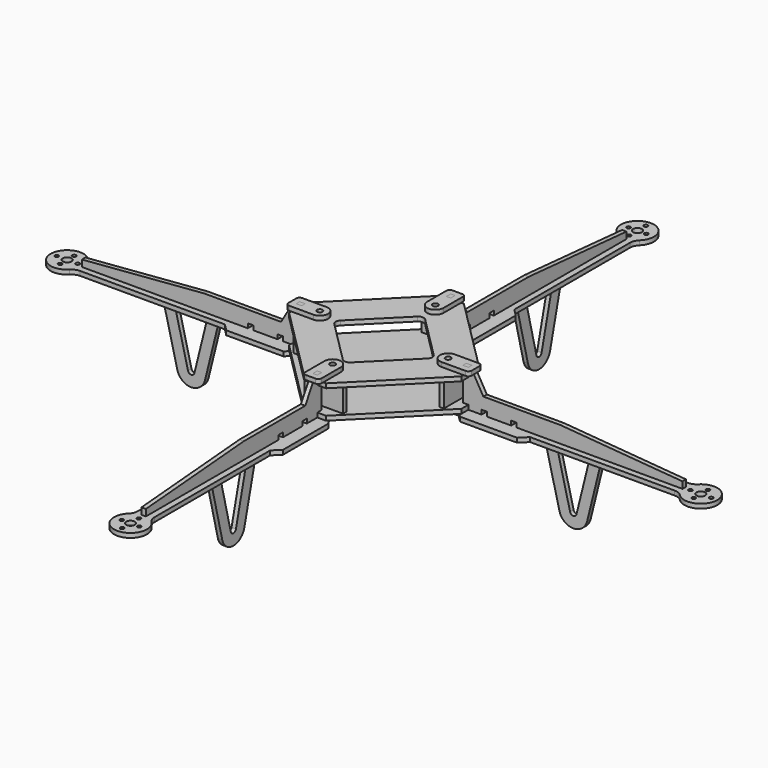
from build123d import *

# Parameters (mm, degrees)
F3_DEPTH  = 4
F7_DEPTH  = 25
F8_R      = 5
F9_R      = 2.5
F9_R_2    = 1.75
F9_R_3    = 4
F11_DEPTH = 4
F13_DEPTH = 2
F15_DEPTH = 2
F16_R     = 2.5
F17_DEPTH = 4
F20_W     = 35
F20_H     = 4
F21_DEPTH = 22
F22_COUNT = 4


# Not quite as in the source:
# - a feature names something its author has since deleted; it is built from what else it names


with BuildPart() as f3:
    # F2 (on Top) → F3 (new body)
    with BuildSketch(Plane.XY):
        Polygon((78.3883476483, 10), (10, 78.3883476483), (2, 78.3883476483), (2, 73.3883476483), (-2, 73.3883476483), (-2, 78.3883476483), (-10, 78.3883476483), (-78.3883476483, 10), (-78.3883476483, 2), (-73.3883476483, 2), (-73.3883476483, -2), (-78.3883476483, -2), (-78.3883476483, -10), (-10, -78.3883476483), (-2, -78.3883476483), (-2, -73.3883476483), (2, -73.3883476483), (2, -78.3883476483), (10, -78.3883476483), (78.3883476483, -10), (78.3883476483, -2), (73.3883476483, -2), (73.3883476483, 2), (78.3883476483, 2), align=None)
    extrude(amount=F3_DEPTH)


with BuildPart() as f5_1:
    # F5: copy of F3
    add(f3.part.moved(Location((0, 0, 26))))

    # F6 (on face) → F7 (cut)
    with BuildSketch(Plane.XY.offset(30)):
        Polygon((-45.9619407771, 0), (0, -45.9619407771), (45.9619407771, 0), (0, 45.9619407771), align=None)
    extrude(amount=-F7_DEPTH, mode=Mode.SUBTRACT)

    # F8
    f8_edges = [f5_1.edges().sort_by_distance(p)[0] for p in [
        (0, -45.961941, 28),
        (-45.961941, 0, 28),
        (0, 45.961941, 28),
        (45.961941, 0, 28),
    ]]
    fillet(f8_edges, radius=F8_R)


with BuildPart() as f11:
    # F9 (on Top) → F11 (new body)
    with BuildSketch(Plane.XY):
        with BuildLine():
            ThreePointArc((7.5, 270.534776577), (8.2804555427, 274.4077599232), (10.5, 277.6762050055))
            ThreePointArc((10.5, 277.6762050055), (0, 303.3883476483), (-10.5, 277.6762050055))
            ThreePointArc((-10.5, 277.6762050055), (-8.2804555427, 274.4077599232), (-7.5, 270.534776577))
            Line((-7.5, 270.534776577), (-7.5, 138.8883476483))
            Line((-7.5, 138.8883476483), (-14, 132.3883476483))
            Line((-14, 132.3883476483), (-14, 80.3883476483))
            Line((-14, 80.3883476483), (-7.5, 73.8883476483))
            Line((-7.5, 73.8883476483), (-7.5, 58.3883476483))
            ThreePointArc((-7.5, 58.3883476483), (0, 50.8883476483), (7.5, 58.3883476483))
            Line((7.5, 58.3883476483), (7.5, 73.8883476483))
            Line((7.5, 73.8883476483), (14, 80.3883476483))
            Line((14, 80.3883476483), (14, 132.3883476483))
            Line((14, 132.3883476483), (7.5, 138.8883476483))
            Line((7.5, 138.8883476483), (7.5, 270.534776577))
        make_face()
        with Locations((0, 58.3883476483)):
            Circle(F9_R, mode=Mode.SUBTRACT)
        with Locations((-8, 288.3883476483)):
            Circle(F9_R_2, mode=Mode.SUBTRACT)
        with Locations((0, 278.8883476483)):
            Circle(F9_R_2, mode=Mode.SUBTRACT)
        with Locations((0, 288.3883476483)):
            Circle(F9_R_3, mode=Mode.SUBTRACT)
        with Locations((0, 297.8883476483)):
            Circle(F9_R_2, mode=Mode.SUBTRACT)
        with Locations((8, 288.3883476483)):
            Circle(F9_R_2, mode=Mode.SUBTRACT)
    extrude(amount=-F11_DEPTH)


with BuildPart() as f13:
    # F12 (on Right) → F13 (new body, symmetric)
    with BuildSketch(Plane.YZ):
        Polygon((162.0486016862, 15), (92.0486016862, 15), (83.3883476483, 30), (78.3883476483, 30), (78.3883476483, 34), (73.3883476483, 34), (73.3883476483, 0), (80.3883476483, 0), (80.3883476483, -4), (90.3883476483, -4), (90.3883476483, 4), (95.3883476483, 4), (95.3883476483, 0), (117.3883476483, 0), (117.3883476483, 4), (122.3883476483, 4), (122.3883476483, 0), (263.3883476483, 0), (263.3883476483, -4), (273.3883476483, -4), (273.3883476483, 6), align=None)
    extrude(amount=F13_DEPTH, both=True)


with BuildPart() as f15:
    # F14 (on Right) → F15 (new body, symmetric)
    with BuildSketch(Plane.YZ):
        with BuildLine():
            Line((154.1888916965, -4), (148.8883476483, -4))
            Line((148.8883476483, -4), (161.2676550527, -54.1173896785))
            ThreePointArc((161.2676550527, -54.1173896785), (173.8883476483, -64), (186.5090402439, -54.1173896785))
            Line((186.5090402439, -54.1173896785), (198.8883476483, -4))
            Line((198.8883476483, -4), (193.5878036001, -4))
            Line((193.5878036001, -4), (193.5878036001, 0))
            Line((193.5878036001, 0), (188.5878036001, 0))
            Line((188.5878036001, 0), (188.5878036001, -4))
            Line((188.5878036001, -4), (176.8008151704, -51.7193976181))
            ThreePointArc((176.8008151704, -51.7193976181), (173.8883476483, -54), (170.9758801263, -51.7193976181))
            Line((170.9758801263, -51.7193976181), (159.1888916965, -4))
            Line((159.1888916965, -4), (159.1888916965, 0))
            Line((159.1888916965, 0), (154.1888916965, 0))
            Line((154.1888916965, 0), (154.1888916965, -4))
        make_face()
    extrude(amount=F15_DEPTH, both=True)


with BuildPart() as f17:
    # F16 (on offset) → F17 (new body)
    with BuildSketch(Plane.XY.offset(30)):
        with BuildLine():
            Line((-7.5, 80.3883476483), (-7.5, 73.8883476483))
            Line((-7.5, 73.8883476483), (-7.5, 58.3883476483))
            ThreePointArc((-7.5, 58.3883476483), (0, 50.8883476483), (7.5, 58.3883476483))
            Line((7.5, 58.3883476483), (7.5, 73.8883476483))
            Line((7.5, 73.8883476483), (7.5, 80.3883476483))
            ThreePointArc((7.5, 80.3883476483), (6.6213203436, 82.5096679919), (4.5, 83.3883476483))
            Line((4.5, 83.3883476483), (-4.5, 83.3883476483))
            ThreePointArc((-4.5, 83.3883476483), (-6.6213203436, 82.5096679919), (-7.5, 80.3883476483))
        make_face()
        with Locations((0, 58.3883476483)):
            Circle(F16_R, mode=Mode.SUBTRACT)
    extrude(amount=F17_DEPTH)

    # F18: cut F13
    add(f13.part, mode=Mode.SUBTRACT)


with BuildPart() as f3_1:
    add(f3.part)

    # F18: cut F13
    add(f13.part, mode=Mode.SUBTRACT)


with BuildPart() as f11_1:
    add(f11.part)

    # F19: cut F13, F15
    add(f13.part, mode=Mode.SUBTRACT)
    add(f15.part, mode=Mode.SUBTRACT)


with BuildPart() as f21:
    # F20 (on face) → F21 (new body, through all)
    with BuildSketch(Plane.XY.offset(4)):
        with Locations((0, 66.3883476483)):
            Rectangle(F20_W, F20_H)
    extrude(amount=F21_DEPTH)


with BuildPart() as f22_1:
    # F22: instance of F17
    add(f17.part.rotate(Axis((0, 0, 50), (0, 0, 1)), 1 * 360 / F22_COUNT))


with BuildPart() as f22_2:
    # F22: instance of F17
    add(f17.part.rotate(Axis((0, 0, 50), (0, 0, 1)), 2 * 360 / F22_COUNT))


with BuildPart() as f22_3:
    # F22: instance of F17
    add(f17.part.rotate(Axis((0, 0, 50), (0, 0, 1)), 3 * 360 / F22_COUNT))


with BuildPart() as f22_4:
    # F22: instance of F15
    add(f15.part.rotate(Axis((0, 0, 50), (0, 0, 1)), 1 * 360 / F22_COUNT))


with BuildPart() as f22_5:
    # F22: instance of F15
    add(f15.part.rotate(Axis((0, 0, 50), (0, 0, 1)), 2 * 360 / F22_COUNT))


with BuildPart() as f22_6:
    # F22: instance of F15
    add(f15.part.rotate(Axis((0, 0, 50), (0, 0, 1)), 3 * 360 / F22_COUNT))


with BuildPart() as f22_7:
    # F22: instance of F13
    add(f13.part.rotate(Axis((0, 0, 50), (0, 0, 1)), 1 * 360 / F22_COUNT))


with BuildPart() as f22_8:
    # F22: instance of F13
    add(f13.part.rotate(Axis((0, 0, 50), (0, 0, 1)), 2 * 360 / F22_COUNT))


with BuildPart() as f22_9:
    # F22: instance of F13
    add(f13.part.rotate(Axis((0, 0, 50), (0, 0, 1)), 3 * 360 / F22_COUNT))


with BuildPart() as f22_10:
    # F22: instance of F11
    add(f11_1.part.rotate(Axis((0, 0, 50), (0, 0, 1)), 1 * 360 / F22_COUNT))


with BuildPart() as f22_11:
    # F22: instance of F11
    add(f11_1.part.rotate(Axis((0, 0, 50), (0, 0, 1)), 2 * 360 / F22_COUNT))


with BuildPart() as f22_12:
    # F22: instance of F11
    add(f11_1.part.rotate(Axis((0, 0, 50), (0, 0, 1)), 3 * 360 / F22_COUNT))


with BuildPart() as f22_13:
    # F22: instance of F21
    add(f21.part.rotate(Axis((0, 0, 50), (0, 0, 1)), 1 * 360 / F22_COUNT))


with BuildPart() as f22_14:
    # F22: instance of F21
    add(f21.part.rotate(Axis((0, 0, 50), (0, 0, 1)), 2 * 360 / F22_COUNT))


with BuildPart() as f22_15:
    # F22: instance of F21
    add(f21.part.rotate(Axis((0, 0, 50), (0, 0, 1)), 3 * 360 / F22_COUNT))


solid = Compound([f5_1.part, f13.part, f15.part, f17.part, f3_1.part, f11_1.part, f21.part, f22_1.part, f22_2.part, f22_3.part, f22_4.part, f22_5.part, f22_6.part, f22_7.part, f22_8.part, f22_9.part, f22_10.part, f22_11.part, f22_12.part, f22_13.part, f22_14.part, f22_15.part])
